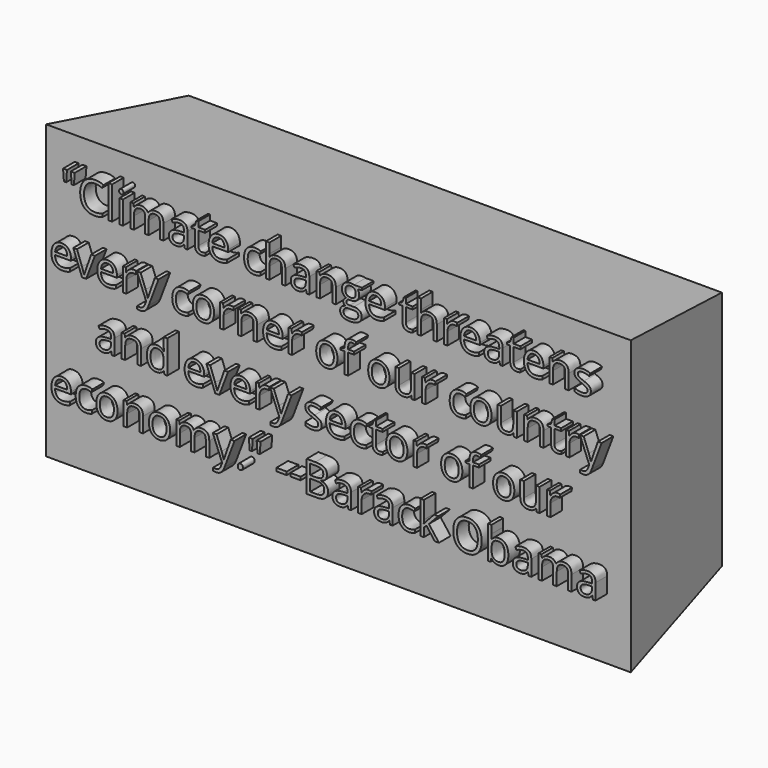
from build123d import *

# Parameters (mm, degrees)
F0_W         = 101.6
F0_H         = 50.8
F1_DEPTH     = 25.4
F1_TAPER     = 10
F2_TEXT_SIZE = 7.5100968962
F3_DEPTH     = 2.54


# Not quite as in the source:
# - Text() gives the source's letters only with a copy of the font that has no kerning and outlines rounded to 1/6400 em; it was checked with that copy


with BuildPart() as f1:
    # F0 (on Front) → F1 (new body)
    with BuildSketch(Plane.XZ):
        with Locations((-50.8, 25.4)):
            Rectangle(F0_W, F0_H)
    extrude(amount=-F1_DEPTH, taper=F1_TAPER)

    # F2 (on face) → F3 (join)
    with BuildSketch(Plane.XZ):
        with Locations((-97.1085482596, 41.3246807493)):
            Text('"Climate change threatens', F2_TEXT_SIZE, font='Open Sans', text_align=(TextAlign.LEFT, TextAlign.BOTTOM))
        with Locations((-99.06, 31.1109489705)):
            Text('every corner of our country', F2_TEXT_SIZE, font='Open Sans', text_align=(TextAlign.LEFT, TextAlign.BOTTOM))
        with Locations((-91.2541930386, 20.8972171917)):
            Text('and every sector of our', F2_TEXT_SIZE, font='Open Sans', text_align=(TextAlign.LEFT, TextAlign.BOTTOM))
        with Locations((-99.06, 10.6834854129)):
            Text('economy." --Barack Obama', F2_TEXT_SIZE, font='Open Sans', text_align=(TextAlign.LEFT, TextAlign.BOTTOM))
    extrude(amount=F3_DEPTH)


solid = f1.part
